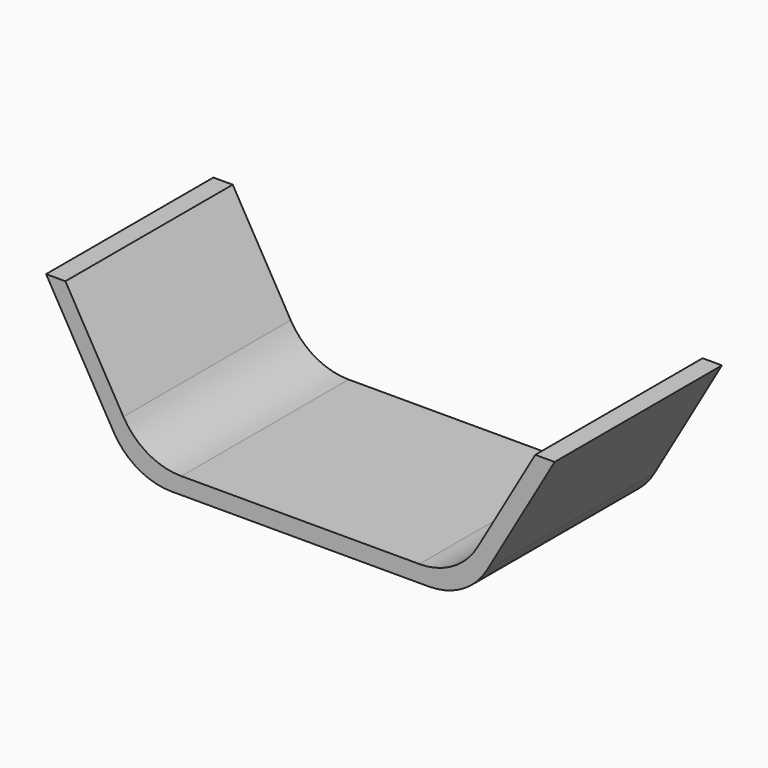
from build123d import *

# Parameters (mm, degrees)
F0_W     = 400
F0_H     = 250
F1_DEPTH = 20
F3_DEPTH = 250
F4_R     = 80


# Not quite as in the source:
# - a pattern or mirror of a feature is missing from the dataset's text; its kind, count and spacing are read off the source's solid


with BuildPart() as f1:
    # F0 (on Top) → F1 (new body)
    with BuildSketch(Plane.XY):
        Rectangle(F0_W, F0_H)
    extrude(amount=F1_DEPTH)

    # F2 (on face) → F3 (join, through all)
    with BuildSketch(Plane.XZ.offset(125)):
        Polygon((-303.9230484541, 180), (-200, 0), (-188.4529946162, 20), (-280.8290376865, 180), align=None)
    f3 = extrude(amount=-F3_DEPTH)

    # F3_copies: F3 across plane
    add(f3.mirror(Plane(origin=(0, 0, 0), x_dir=(0, 0, 1), z_dir=(1, 0, 0))))

    # F4
    f4_edges = [f1.edges().sort_by_distance(p)[0] for p in [
        (-188.452995, 0, 20),
        (-200, 0, 0),
        (188.452995, 0, 20),
        (200, 0, 0),
    ]]
    fillet(f4_edges, radius=F4_R)


solid = f1.part
